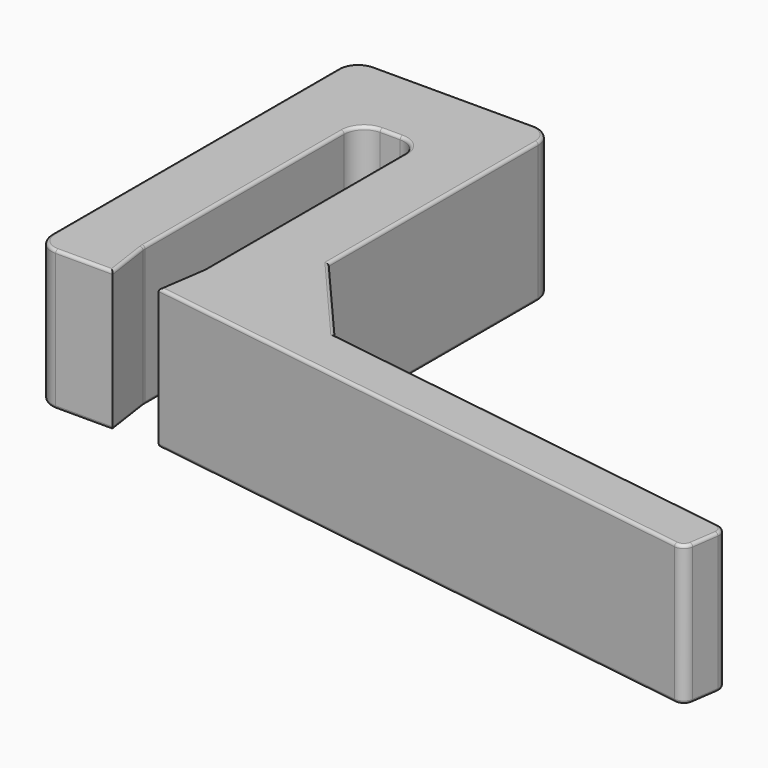
from build123d import *

# Parameters (mm, degrees)
F1_DEPTH     = 14
F2_R         = 2
F3_W         = 4.692493906
F3_H         = 14
F4_DEPTH     = 60
F5_SIZE      = 8
F6_R         = 0.3
F7_T1_DEPTH  = 14
F7_T4_ANGLE  = 90
F7_T6_ANGLE  = 90
F7_T8_ANGLE  = 90
F7_T10_ANGLE = 90


# Not quite as in the source:
# - a fillet or chamfer that OpenCascade refuses, or shapes differently, is made with other operations: its cross-section is extruded or revolved along the edge and cut away or added
# - a feature names something its author has since deleted; it is built from what else it names


with BuildPart() as f1:
    # F0 (on Top) → F1 (new body)
    with BuildSketch(Plane.XY):
        Polygon((0, 27), (0, 0), (-0.7, -4.7870394774), (7, -4.7870394774), (7, 35), (-13, 35), (-13, -4.7870394774), (-5.3, -4.7870394774), (-6, 0), (-6, 27), align=None)
    extrude(amount=F1_DEPTH)

    # F2
    f2_edges = [f1.edges().sort_by_distance(p)[0] for p in [
        (-13, 35, 7),
        (-13, -4.787039, 7),
        (0, 27, 7),
        (0, 0, 7),
        (7, 35, 7),
        (-6, 0, 7),
        (-6, 27, 7),
    ]]
    fillet(f2_edges, radius=F2_R)

    # F3 (on face) → F4 (join)
    with BuildSketch(Plane(origin=(0, 0, 0), x_dir=(-0.1446894238, -0.9894771198, 0), z_dir=(-0.9894771198, 0.1446894238, 0))):
        with Locations((2.4917016782, 7)):
            Rectangle(F3_W, F3_H)
    extrude(amount=-F4_DEPTH)

    # F5
    f5_edges = [f1.edges().sort_by_distance(p)[0] for p in [
        (7, -1.170599, 7),
    ]]
    chamfer(f5_edges, length=F5_SIZE)

    # F6
    f6_edges = [f1.edges().sort_by_distance(p)[0] for p in [
        (37.131699, -5.576702, 14),
        (10.957908, 2.250644, 14),
        (59.008104, -11.146847, 14),
        (7, 19.914701, 14),
        (28.984314, -9.127722, 14),
        (6.414214, 34.414214, 14),
        (-0.360523, -2.465482, 14),
        (-3, 35, 14),
        (-0.005268, 0.000383, 14),
        (-12.414214, 34.414214, 14),
        (0, 12.572727, 14),
        (-13, 15.10648, 14),
        (-0.585786, 26.414214, 14),
        (-12.414214, -4.201253, 14),
        (-3, 27, 14),
        (-8.15, -4.787039, 14),
        (-5.414214, 26.414214, 14),
        (-5.639477, -2.465482, 14),
        (-6, 12.572727, 14),
        (-5.994732, 0.000383, 14),
        (37.131699, -5.576702, 0),
        (10.957908, 2.250644, 0),
        (59.008104, -11.146847, 0),
        (7, 19.914701, 0),
        (28.984314, -9.127722, 0),
        (6.414214, 34.414214, 0),
        (-0.360523, -2.465482, 0),
        (-3, 35, 0),
        (-0.005268, 0.000383, 0),
        (-12.414214, 34.414214, 0),
        (0, 12.572727, 0),
        (-13, 15.10648, 0),
        (-0.585786, 26.414214, 0),
        (-12.414214, -4.201253, 0),
        (-3, 27, 0),
        (-8.15, -4.787039, 0),
        (-5.414214, 26.414214, 0),
        (-5.639477, -2.465482, 0),
        (-6, 12.572727, 0),
        (-5.994732, 0.000383, 0),
    ]]
    fillet(f6_edges, radius=F6_R)

    # F7: fillet of radius 1 on 2 edges, made by hand

    # F7_s2 → F7_t1 (cut)
    with BuildSketch(Plane.XY):
        with BuildLine():
            ThreePointArc((58.3581043085, -8.6806001289), (59.0153917386, -9.0727221402), (59.2028920045, -9.8147666726))
            Line((59.2028920045, -9.8147666726), (59.3475814283, -8.8252895527))
            Line((59.3475814283, -8.8252895527), (58.3581043085, -8.6806001289))
        make_face()
        with BuildLine():
            ThreePointArc((58.8133166125, -12.4789277878), (58.4211946012, -13.136215218), (57.6791500689, -13.3237154838))
            Line((57.6791500689, -13.3237154838), (58.6686271887, -13.4684049076))
            Line((58.6686271887, -13.4684049076), (58.8133166125, -12.4789277878))
        make_face()
    extrude(amount=F7_T1_DEPTH, mode=Mode.SUBTRACT)

    # F7_s3 → F7_t4 (revolve, cut)
    with BuildSketch(Plane(origin=(-0.5553105762, -3.7975623576, 0), x_dir=(0, 0, 1), z_dir=(0.1446894238, 0.9894771198, 0))):
        with BuildLine():
            ThreePointArc((0, 59.7), (0.0878679656, 59.9121320344), (0.3, 60))
            Line((0.3, 60), (0, 60))
            Line((0, 60), (0, 59.7))
        make_face()
    revolve(axis=Axis((57.8238394927, -12.334238364, 0), (0, 0, -1)), revolution_arc=F7_T4_ANGLE, mode=Mode.SUBTRACT)

    # F7_s5 → F7_t6 (revolve, cut)
    with BuildSketch(Plane(origin=(58.3791500689, -8.5366760064, 0), x_dir=(0, 0, 1), z_dir=(-0.9894771198, 0.1446894238, 0))):
        with BuildLine():
            ThreePointArc((14, -4.5379486312), (13.9121320344, -4.7500806655), (13.7, -4.8379486312))
            Line((13.7, -4.8379486312), (14, -4.8379486312))
            Line((14, -4.8379486312), (14, -4.5379486312))
        make_face()
    revolve(axis=Axis((57.8238394927, -12.334238364, 14), (0, 0, 1)), revolution_arc=F7_T6_ANGLE, mode=Mode.SUBTRACT)

    # F7_s7 → F7_t8 (revolve, cut)
    with BuildSketch(Plane(origin=(-0.1657351842, -1.1334012423, 0), x_dir=(0, 0, 1), z_dir=(-0.1446894238, -0.9894771198, 0))):
        with BuildLine():
            ThreePointArc((14, -59.7), (13.9121320344, -59.9121320344), (13.7, -60))
            Line((13.7, -60), (14, -60))
            Line((14, -60), (14, -59.7))
        make_face()
    revolve(axis=Axis((58.2134148846, -9.6700772487, 14), (0, 0, 1)), revolution_arc=F7_T8_ANGLE, mode=Mode.SUBTRACT)

    # F7_s9 → F7_t10 (revolve, cut)
    with BuildSketch(Plane(origin=(58.3791500689, -8.5366760064, 0), x_dir=(0, 0, 1), z_dir=(-0.9894771198, 0.1446894238, 0))):
        with BuildLine():
            ThreePointArc((0, -0.4454547252), (0.0878679656, -0.2333226908), (0.3, -0.1454547252))
            Line((0.3, -0.1454547252), (0, -0.1454547252))
            Line((0, -0.1454547252), (0, -0.4454547252))
        make_face()
    revolve(axis=Axis((58.2134148846, -9.6700772487, 0), (0, 0, -1)), revolution_arc=F7_T10_ANGLE, mode=Mode.SUBTRACT)


solid = f1.part
